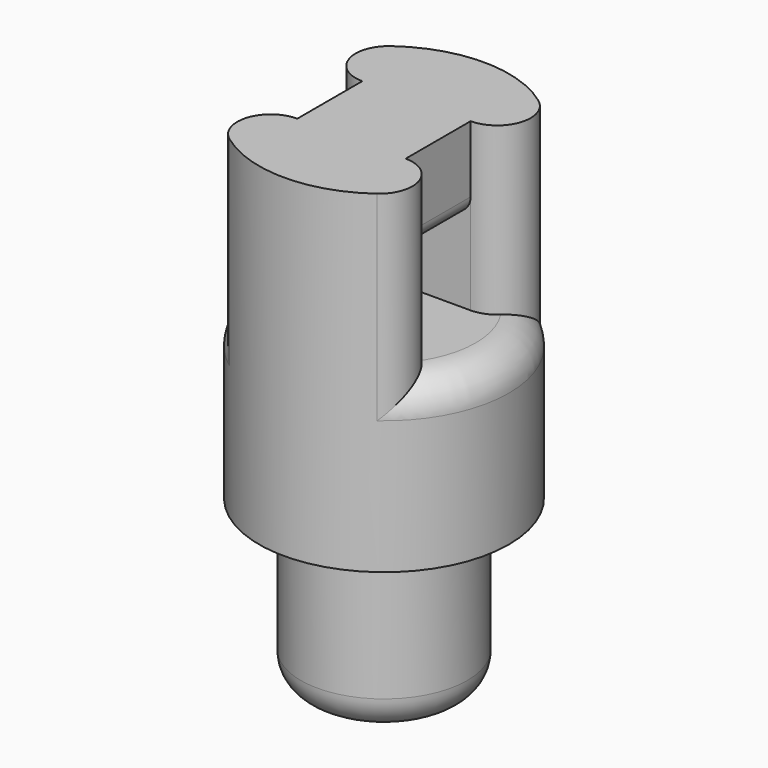
from build123d import *

# Parameters (mm, degrees)
F0_R         = 5
F1_DEPTH     = 10
F2_R         = 7.5
F2_R_2       = 5
F3_DEPTH     = 15
F5_DEPTH     = 5
F6_T1_DEPTH  = 16.216012475
F6_T6_ANGLE  = 57.151354628
F6_T11_ANGLE = 114.30679143
F6_T17_ANGLE = 57.151354628
F6_T23_ANGLE = 57.151354628
F6_T27_DEPTH = 27.4320249501
F6_T34_DEPTH = 27.4320249501
F6_T38_ANGLE = 114.30679143
F6_T45_ANGLE = 114.30679143
F6_T49_DEPTH = 27.4320249501
F6_T56_DEPTH = 27.4320249501
F6_T60_ANGLE = 57.151354628
F7_R         = 2
F8_DEPTH     = 5
F9_W         = 6.5028829414
F9_H         = 5
F10_DEPTH    = 6
F11_R        = 1


# Not quite as in the source:
# - a fillet or chamfer that OpenCascade refuses, or shapes differently, is made with other operations: its cross-section is extruded or revolved along the edge and cut away or added


with BuildPart() as f1:
    # F0 (on Top) → F1 (new body)
    with BuildSketch(Plane.XY):
        Circle(F0_R)
    extrude(amount=F1_DEPTH)

    # F2 (on face) → F3 (join)
    with BuildSketch(Plane.XY.offset(10)):
        Circle(F2_R)
        Circle(F2_R_2, mode=Mode.SUBTRACT)
        Circle(F2_R_2)
    extrude(amount=F3_DEPTH)

    # F4 (on face) → F5 (cut)
    with BuildSketch(Plane.XY.offset(25)):
        with BuildLine():
            Line((-10.1172067225, -2.4360036477), (-7.0933691733, -2.4360036477))
            ThreePointArc((-7.0933691733, -2.4360036477), (-7.5, 0), (-7.0933691733, 2.4360036477))
            Line((-7.0933691733, 2.4360036477), (-10.1172067225, 2.4360036477))
            Line((-10.1172067225, 2.4360036477), (-10.1172067225, -2.4360036477))
        make_face()
        with BuildLine():
            Line((-7.0933691733, -2.4360036477), (7.0933691733, -2.4360036477))
            ThreePointArc((7.0933691733, -2.4360036477), (7.3976438411, -1.2348544855), (7.5, 0))
            ThreePointArc((7.5, 0), (7.3976438411, 1.2348544855), (7.0933691733, 2.4360036477))
            Line((7.0933691733, 2.4360036477), (-7.0933691733, 2.4360036477))
            ThreePointArc((-7.0933691733, 2.4360036477), (-7.5, 0), (-7.0933691733, -2.4360036477))
        make_face()
        with BuildLine():
            Line((7.0933691733, -2.4360036477), (10.1172067225, -2.4360036477))
            Line((10.1172067225, -2.4360036477), (10.1172067225, 2.4360036477))
            Line((10.1172067225, 2.4360036477), (7.0933691733, 2.4360036477))
            ThreePointArc((7.0933691733, 2.4360036477), (7.3976438411, 1.2348544855), (7.5, 0))
            ThreePointArc((7.5, 0), (7.3976438411, -1.2348544855), (7.0933691733, -2.4360036477))
        make_face()
    extrude(amount=-F5_DEPTH, mode=Mode.SUBTRACT)

    # F6: fillet of radius 2 on 7 edges, made by hand

    # F6_s2 → F6_t1 (cut)
    with BuildSketch(Plane.XY.offset(20)):
        with BuildLine():
            ThreePointArc((-4.4337838236, 6.0490958833), (-5.1522550427, 3.8139845448), (-3.2514414707, 2.4360036477))
            Line((-3.2514414707, 2.4360036477), (-7.0933691733, 2.4360036477))
            ThreePointArc((-7.0933691733, 2.4360036477), (-6.0400681229, 4.4460743438), (-4.4337838236, 6.0490958833))
        make_face()
        with BuildLine():
            ThreePointArc((4.4337838236, 6.0490958833), (5.1522550427, 3.8139845448), (3.2514414707, 2.4360036477))
            Line((3.2514414707, 2.4360036477), (7.0933691733, 2.4360036477))
            ThreePointArc((7.0933691733, 2.4360036477), (6.0400681229, 4.4460743438), (4.4337838236, 6.0490958833))
        make_face()
        with BuildLine():
            ThreePointArc((4.4337838236, -6.0490958833), (5.1522550427, -3.8139845448), (3.2514414707, -2.4360036477))
            Line((3.2514414707, -2.4360036477), (7.0933691733, -2.4360036477))
            ThreePointArc((7.0933691733, -2.4360036477), (6.0400681229, -4.4460743438), (4.4337838236, -6.0490958833))
        make_face()
        with BuildLine():
            ThreePointArc((-4.4337838236, -6.0490958833), (-5.1522550427, -3.8139845448), (-3.2514414707, -2.4360036477))
            Line((-3.2514414707, -2.4360036477), (-7.0933691733, -2.4360036477))
            ThreePointArc((-7.0933691733, -2.4360036477), (-6.0400681229, -4.4460743438), (-4.4337838236, -6.0490958833))
        make_face()
    extrude(amount=F6_T1_DEPTH, mode=Mode.SUBTRACT)


with BuildPart() as f6_tool4:
    # F6_s5 → F6_t6 (revolve)
    with BuildSketch(Plane.XZ):
        with BuildLine():
            ThreePointArc((7.5, 18), (6.9142135624, 19.4142135624), (5.5, 20))
            Line((5.5, 20), (7.5, 20))
            Line((7.5, 20), (7.5, 18))
        make_face()
    revolve(axis=Axis((0, 0, 20), (0, 0, -1)), revolution_arc=F6_T6_ANGLE)

    split(bisect_by=Plane.XZ.offset(2.4360036477), keep=Keep.BOTTOM)


with BuildPart() as f1_1:
    add(f1.part)

    # F6_t3: cut F6_tool4
    add(f6_tool4.part, mode=Mode.SUBTRACT)


with BuildPart() as f6_tool9:
    # F6_s10 → F6_t11 (revolve)
    with BuildSketch(Plane(origin=(0, 0, 0), x_dir=(0, 0, 1), z_dir=(0.840125701, -0.5423917464, 0))):
        with BuildLine():
            ThreePointArc((18, 7.5), (19.4142135624, 6.9142135624), (20, 5.5))
            Line((20, 5.5), (20, 7.5))
            Line((20, 7.5), (18, 7.5))
        make_face()
    revolve(axis=Axis((0, 0, 20), (0, 0, -1)), revolution_arc=F6_T11_ANGLE)

    split(bisect_by=Plane.XZ.offset(-2.4360036477), keep=Keep.TOP)

    split(bisect_by=Plane.XZ.offset(2.4360036477), keep=Keep.BOTTOM)


with BuildPart() as f1_2:
    add(f1_1.part)

    # F6_t8: cut F6_tool9
    add(f6_tool9.part, mode=Mode.SUBTRACT)


with BuildPart() as f6_tool15:
    # F6_s16 → F6_t17 (revolve)
    with BuildSketch(Plane(origin=(0, 0, 0), x_dir=(0, 0, 1), z_dir=(-0.8401063785, 0.5424216744, 0))):
        with BuildLine():
            ThreePointArc((18, 7.5), (19.4142135624, 6.9142135624), (20, 5.5))
            Line((20, 5.5), (20, 7.5))
            Line((20, 7.5), (18, 7.5))
        make_face()
    revolve(axis=Axis((0, 0, 20), (0, 0, -1)), revolution_arc=F6_T17_ANGLE)

    split(bisect_by=Plane.XZ.offset(-2.4360036477), keep=Keep.TOP)


with BuildPart() as f1_3:
    add(f1_2.part)

    # F6_t14: cut F6_tool15
    add(f6_tool15.part, mode=Mode.SUBTRACT)


with BuildPart() as f6_tool21:
    # F6_s22 → F6_t23 (revolve)
    with BuildSketch(Plane.XZ):
        with BuildLine():
            ThreePointArc((7.5, 18), (6.9142135624, 19.4142135624), (5.5, 20))
            Line((5.5, 20), (7.5, 20))
            Line((7.5, 20), (7.5, 18))
        make_face()
    revolve(axis=Axis((0, 0, 20), (0, 0, -1)), revolution_arc=F6_T23_ANGLE)

    split(bisect_by=Plane.XZ.offset(2.4360036477), keep=Keep.TOP)


with BuildPart() as f6_tool25:
    # F6_s26 → F6_t27 (new body)
    with BuildSketch(Plane.XY.offset(36.216012475)):
        with BuildLine():
            ThreePointArc((4.4337838236, -6.0490958833), (5.1522550427, -3.8139845448), (3.2514414707, -2.4360036477))
            Line((3.2514414707, -2.4360036477), (7.0933691733, -2.4360036477))
            ThreePointArc((7.0933691733, -2.4360036477), (6.0400681229, -4.4460743438), (4.4337838236, -6.0490958833))
        make_face()
    extrude(amount=-F6_T27_DEPTH)

    split(bisect_by=Plane.XY.offset(20), keep=Keep.BOTTOM)


with BuildPart() as f6_tool21_1:
    add(f6_tool21.part)

    # F6_t29: intersect F6_tool25
    add(f6_tool25.part, mode=Mode.INTERSECT)


with BuildPart() as f1_4:
    add(f1_3.part)

    # F6_t19: cut F6_tool21
    add(f6_tool21_1.part, mode=Mode.SUBTRACT)


with BuildPart() as f6_tool32:
    # F6_s33 → F6_t34 (new body)
    with BuildSketch(Plane.XY.offset(36.216012475)):
        with BuildLine():
            ThreePointArc((-4.4337838236, -6.0490958833), (-5.1522550427, -3.8139845448), (-3.2514414707, -2.4360036477))
            Line((-3.2514414707, -2.4360036477), (-7.0933691733, -2.4360036477))
            ThreePointArc((-7.0933691733, -2.4360036477), (-6.0400681229, -4.4460743438), (-4.4337838236, -6.0490958833))
        make_face()
    extrude(amount=-F6_T34_DEPTH)

    split(bisect_by=Plane.XY.offset(20), keep=Keep.BOTTOM)


with BuildPart() as f6_tool36:
    # F6_s37 → F6_t38 (revolve)
    with BuildSketch(Plane(origin=(0, 0, 0), x_dir=(0, 0, 1), z_dir=(0.840125701, -0.5423917464, 0))):
        with BuildLine():
            ThreePointArc((18, 7.5), (19.4142135624, 6.9142135624), (20, 5.5))
            Line((20, 5.5), (20, 7.5))
            Line((20, 7.5), (18, 7.5))
        make_face()
    revolve(axis=Axis((0, 0, 20), (0, 0, -1)), revolution_arc=F6_T38_ANGLE)

    split(bisect_by=Plane.XZ.offset(2.4360036477), keep=Keep.TOP)


with BuildPart() as f6_tool32_1:
    add(f6_tool32.part)

    # F6_t40: intersect F6_tool36
    add(f6_tool36.part, mode=Mode.INTERSECT)


with BuildPart() as f1_5:
    add(f1_4.part)

    # F6_t30: cut F6_tool32
    add(f6_tool32_1.part, mode=Mode.SUBTRACT)


with BuildPart() as f6_tool43:
    # F6_s44 → F6_t45 (revolve)
    with BuildSketch(Plane(origin=(0, 0, 0), x_dir=(0, 0, 1), z_dir=(0.840125701, -0.5423917464, 0))):
        with BuildLine():
            ThreePointArc((18, 7.5), (19.4142135624, 6.9142135624), (20, 5.5))
            Line((20, 5.5), (20, 7.5))
            Line((20, 7.5), (18, 7.5))
        make_face()
    revolve(axis=Axis((0, 0, 20), (0, 0, -1)), revolution_arc=F6_T45_ANGLE)

    split(bisect_by=Plane.XZ.offset(-2.4360036477), keep=Keep.BOTTOM)


with BuildPart() as f6_tool47:
    # F6_s48 → F6_t49 (new body)
    with BuildSketch(Plane.XY.offset(36.216012475)):
        with BuildLine():
            ThreePointArc((-4.4337838236, 6.0490958833), (-5.1522550427, 3.8139845448), (-3.2514414707, 2.4360036477))
            Line((-3.2514414707, 2.4360036477), (-7.0933691733, 2.4360036477))
            ThreePointArc((-7.0933691733, 2.4360036477), (-6.0400681229, 4.4460743438), (-4.4337838236, 6.0490958833))
        make_face()
    extrude(amount=-F6_T49_DEPTH)

    split(bisect_by=Plane.XY.offset(20), keep=Keep.BOTTOM)


with BuildPart() as f6_tool43_1:
    add(f6_tool43.part)

    # F6_t51: intersect F6_tool47
    add(f6_tool47.part, mode=Mode.INTERSECT)


with BuildPart() as f1_6:
    add(f1_5.part)

    # F6_t41: cut F6_tool43
    add(f6_tool43_1.part, mode=Mode.SUBTRACT)


with BuildPart() as f6_tool54:
    # F6_s55 → F6_t56 (new body)
    with BuildSketch(Plane.XY.offset(36.216012475)):
        with BuildLine():
            ThreePointArc((4.4337838236, 6.0490958833), (5.1522550427, 3.8139845448), (3.2514414707, 2.4360036477))
            Line((3.2514414707, 2.4360036477), (7.0933691733, 2.4360036477))
            ThreePointArc((7.0933691733, 2.4360036477), (6.0400681229, 4.4460743438), (4.4337838236, 6.0490958833))
        make_face()
    extrude(amount=-F6_T56_DEPTH)

    split(bisect_by=Plane.XY.offset(20), keep=Keep.BOTTOM)


with BuildPart() as f6_tool58:
    # F6_s59 → F6_t60 (revolve)
    with BuildSketch(Plane(origin=(0, 0, 0), x_dir=(0, 0, 1), z_dir=(-0.8401063785, 0.5424216744, 0))):
        with BuildLine():
            ThreePointArc((18, 7.5), (19.4142135624, 6.9142135624), (20, 5.5))
            Line((20, 5.5), (20, 7.5))
            Line((20, 7.5), (18, 7.5))
        make_face()
    revolve(axis=Axis((0, 0, 20), (0, 0, -1)), revolution_arc=F6_T60_ANGLE)

    split(bisect_by=Plane.XZ.offset(-2.4360036477), keep=Keep.BOTTOM)


with BuildPart() as f6_tool54_1:
    add(f6_tool54.part)

    # F6_t62: intersect F6_tool58
    add(f6_tool58.part, mode=Mode.INTERSECT)


with BuildPart() as f1_7:
    add(f1_6.part)

    # F6_t52: cut F6_tool54
    add(f6_tool54_1.part, mode=Mode.SUBTRACT)

    # F7
    f7_edges = [f1_7.edges().sort_by_distance(p)[0] for p in [
        (-5, 0, 0),
    ]]
    fillet(f7_edges, radius=F7_R)

    # F8 (add): faces of the model
    f8_faces = [f1_7.faces().sort_by_distance(p)[0] for p in [
        (0, 4.7439045523, 25),
        (0, -4.7439045523, 25),
    ]]
    extrude(f8_faces, amount=F8_DEPTH)

    # F9 (on face) → F10 (join)
    with BuildSketch(Plane.XZ.offset(-2.4360036477)):
        with Locations((0, 27.5)):
            Rectangle(F9_W, F9_H)
    extrude(amount=F10_DEPTH)

    # F11
    f11_edges = [f1_7.edges().sort_by_distance(p)[0] for p in [
        (3.251441, 0, 25),
        (-3.251441, 0, 25),
    ]]
    fillet(f11_edges, radius=F11_R)


solid = f1_7.part
